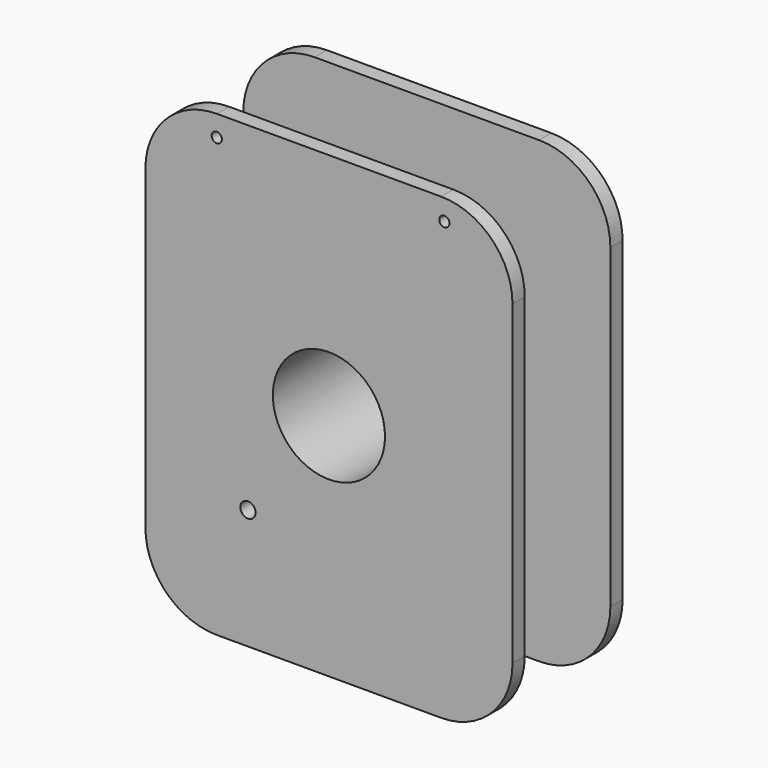
from build123d import *

# Parameters (mm, degrees)
F0_W      = 36
F0_H      = 45
F0_R      = 5.5
F1_DEPTH  = 1.5
F2_W      = 19
F2_H      = 24
F2_R      = 5.5
F3_DEPTH  = 12
F4_W      = 36
F4_H      = 45
F4_W_2    = 19
F4_H_2    = 24
F4_R      = 5.5
F5_DEPTH  = 1.5
F6_R      = 7
F7_R      = 0.75
F8_DEPTH  = 2.5
F9_R      = 0.5
F10_DEPTH = 2.5


# Not quite as in the source:
# - a feature names something its author has since deleted; it is built from what else it names


with BuildPart() as f1:
    # F0 (on Front) → F1 (new body)
    with BuildSketch(Plane.XZ):
        Rectangle(F0_W, F0_H)
        Circle(F0_R, mode=Mode.SUBTRACT)
    extrude(amount=F1_DEPTH)

    # F2 (on face) → F3 (join)
    with BuildSketch(Plane.XZ.offset(1.5)):
        Rectangle(F2_W, F2_H)
        Circle(F2_R, mode=Mode.SUBTRACT)
    extrude(amount=F3_DEPTH)

    # F4 (on face) → F5 (join)
    with BuildSketch(Plane.XZ.offset(13.5)):
        Rectangle(F4_W, F4_H)
        Rectangle(F4_W_2, F4_H_2, mode=Mode.SUBTRACT)
        Rectangle(F4_W_2, F4_H_2)
        Circle(F4_R, mode=Mode.SUBTRACT)
    extrude(amount=-F5_DEPTH)

    # F6
    f6_edges = [f1.edges().sort_by_distance(p)[0] for p in [
        (9.5, -6.75, 12),
        (9.5, -6.75, -12),
        (18, -0.75, 22.5),
        (18, -12.75, 22.5),
        (18, -12.75, -22.5),
        (18, -0.75, -22.5),
        (-18, -0.75, -22.5),
        (-18, -12.75, -22.5),
        (-9.5, -6.75, -12),
        (-9.5, -6.75, 12),
        (-18, -0.75, 22.5),
        (-18, -12.75, 22.5),
    ]]
    fillet(f6_edges, radius=F6_R)

    # F7 (on face) → F8 (cut)
    with BuildSketch(Plane.XZ.offset(13.5)):
        with Locations((-7.9445969313, -10.7102040201)):
            Circle(F7_R)
    extrude(amount=-F8_DEPTH, mode=Mode.SUBTRACT)

    # F9 (on face) → F10 (cut)
    with BuildSketch(Plane.XZ.offset(13.5)):
        with Locations((-11, 20.4497474683)):
            Circle(F9_R)
        with Locations((11.3213816658, 20.4497474683)):
            Circle(F9_R)
    extrude(amount=-F10_DEPTH, mode=Mode.SUBTRACT)


solid = f1.part
